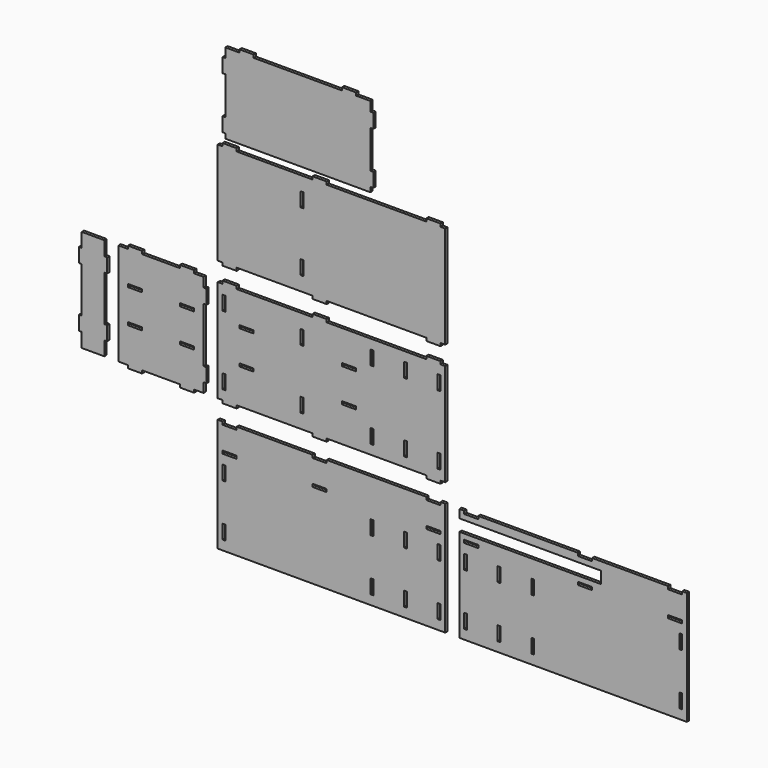
from build123d import *

# Parameters (mm, degrees)
F0_W     = 15.494
F0_H     = 76.2
F0_W_2   = 76.2
F0_H_2   = 15.494
F1_DEPTH = 15.494


# Not quite as in the source:
# - a feature names something its author has since deleted; it is built from what else it names


with BuildPart() as f1:
    # F0 (on Front) → F1 (new body)
    with BuildSketch(Plane.XZ):
        Polygon((1909.7625, -985.8375), (1909.7625, -376.2375), (1884.3625, -376.2375), (1884.3625, -391.7315), (1808.1625, -391.7315), (1808.1625, -376.2375), (1400.175, -376.2375), (1400.175, -391.7315), (1323.975, -391.7315), (1323.975, -376.2375), (788.9875, -376.2375), (788.9875, -391.7315), (712.7875, -391.7315), (712.7875, -376.2375), (687.3875, -376.2375), (687.3875, -420.6875), (1449.3875, -420.6875), (1449.3875, -484.1875), (687.3875, -484.1875), (687.3875, -985.8375), align=None)
        with Locations((720.5345, -896.9375)):
            Rectangle(F0_W, F0_H, mode=Mode.SUBTRACT)
        with Locations((901.1285, -896.9375)):
            Rectangle(F0_W, F0_H, mode=Mode.SUBTRACT)
        with Locations((1081.7225, -896.9375)):
            Rectangle(F0_W, F0_H, mode=Mode.SUBTRACT)
        with Locations((720.5345, -617.5375)):
            Rectangle(F0_W, F0_H, mode=Mode.SUBTRACT)
        with Locations((901.1285, -617.5375)):
            Rectangle(F0_W, F0_H, mode=Mode.SUBTRACT)
        with Locations((1081.7225, -617.5375)):
            Rectangle(F0_W, F0_H, mode=Mode.SUBTRACT)
        with Locations((750.8875, -520.8905)):
            Rectangle(F0_W_2, F0_H_2, mode=Mode.SUBTRACT)
        with Locations((1876.6155, -896.9375)):
            Rectangle(F0_W, F0_H, mode=Mode.SUBTRACT)
        with Locations((1362.075, -520.8905)):
            Rectangle(F0_W_2, F0_H_2, mode=Mode.SUBTRACT)
        with Locations((1876.6155, -617.5375)):
            Rectangle(F0_W, F0_H, mode=Mode.SUBTRACT)
        with Locations((1846.2625, -520.8905)):
            Rectangle(F0_W_2, F0_H_2, mode=Mode.SUBTRACT)
    extrude(amount=F1_DEPTH)


with BuildPart() as f1b:
    # F0 (on Front) → F1, piece 2 (new body)
    with BuildSketch(Plane.XZ):
        Polygon((-585.7875, -376.2375), (-611.1875, -376.2375), (-611.1875, -985.8375), (611.1875, -985.8375), (611.1875, -376.2375), (585.7875, -376.2375), (585.7875, -391.7315), (509.5875, -391.7315), (509.5875, -376.2375), (-25.4, -376.2375), (-25.4, -391.7315), (-101.6, -391.7315), (-101.6, -376.2375), (-509.5875, -376.2375), (-509.5875, -391.7315), (-585.7875, -391.7315), align=None)
        with Locations((-578.0405, -896.9375)):
            Rectangle(F0_W, F0_H, mode=Mode.SUBTRACT)
        with Locations((-578.0405, -617.5375)):
            Rectangle(F0_W, F0_H, mode=Mode.SUBTRACT)
        with Locations((-547.6875, -520.8905)):
            Rectangle(F0_W_2, F0_H_2, mode=Mode.SUBTRACT)
        with Locations((216.8525, -896.9375)):
            Rectangle(F0_W, F0_H, mode=Mode.SUBTRACT)
        with Locations((216.8525, -617.5375)):
            Rectangle(F0_W, F0_H, mode=Mode.SUBTRACT)
        with Locations((-63.5, -520.8905)):
            Rectangle(F0_W_2, F0_H_2, mode=Mode.SUBTRACT)
        with Locations((397.4465, -896.9375)):
            Rectangle(F0_W, F0_H, mode=Mode.SUBTRACT)
        with Locations((578.0405, -896.9375)):
            Rectangle(F0_W, F0_H, mode=Mode.SUBTRACT)
        with Locations((397.4465, -617.5375)):
            Rectangle(F0_W, F0_H, mode=Mode.SUBTRACT)
        with Locations((578.0405, -617.5375)):
            Rectangle(F0_W, F0_H, mode=Mode.SUBTRACT)
        with Locations((547.6875, -520.8905)):
            Rectangle(F0_W_2, F0_H_2, mode=Mode.SUBTRACT)
    extrude(amount=F1_DEPTH)


with BuildPart() as f1c:
    # F0 (on Front) → F1, piece 3 (new body)
    with BuildSketch(Plane.XZ):
        Polygon((585.7875, 376.2375), (611.1875, 376.2375), (611.1875, 925.5125), (585.7875, 925.5125), (509.5875, 925.5125), (-25.4, 925.5125), (-101.6, 925.5125), (-509.5875, 925.5125), (-585.7875, 925.5125), (-611.1875, 925.5125), (-611.1875, 376.2375), (-585.7875, 376.2375), (-509.5875, 376.2375), (-101.6, 376.2375), (-25.4, 376.2375), (509.5875, 376.2375), align=None)
        with Locations((-158.5595, 490.5375)):
            Rectangle(F0_W, F0_H, mode=Mode.SUBTRACT)
        with Locations((-158.5595, 811.2125)):
            Rectangle(F0_W, F0_H, mode=Mode.SUBTRACT)
        with Locations((-547.6875, 368.4905)):
            Rectangle(F0_W_2, F0_H_2)
        with Locations((-63.5, 368.4905)):
            Rectangle(F0_W_2, F0_H_2)
        with Locations((547.6875, 368.4905)):
            Rectangle(F0_W_2, F0_H_2)
        with Locations((547.6875, 933.2595)):
            Rectangle(F0_W_2, F0_H_2)
        with Locations((-63.5, 933.2595)):
            Rectangle(F0_W_2, F0_H_2)
        with Locations((-547.6875, 933.2595)):
            Rectangle(F0_W_2, F0_H_2)
    extrude(amount=F1_DEPTH)


with BuildPart() as f1d:
    # F0 (on Front) → F1, piece 4 (new body)
    with BuildSketch(Plane.XZ):
        Polygon((611.1875, -274.6375), (611.1875, 274.6375), (585.7875, 274.6375), (509.5875, 274.6375), (-25.4, 274.6375), (-101.6, 274.6375), (-509.5875, 274.6375), (-585.7875, 274.6375), (-611.1875, 274.6375), (-611.1875, -274.6375), (-585.7875, -274.6375), (-509.5875, -274.6375), (-101.6, -274.6375), (-25.4, -274.6375), (509.5875, -274.6375), (585.7875, -274.6375), align=None)
        with Locations((-578.0405, -185.7375)):
            Rectangle(F0_W, F0_H, mode=Mode.SUBTRACT)
        with Locations((-578.0405, 185.7375)):
            Rectangle(F0_W, F0_H, mode=Mode.SUBTRACT)
        with Locations((-158.5595, -160.3375)):
            Rectangle(F0_W, F0_H, mode=Mode.SUBTRACT)
        with Locations((216.8525, -185.7375)):
            Rectangle(F0_W, F0_H, mode=Mode.SUBTRACT)
        with Locations((-455.9935, -78.8035)):
            Rectangle(F0_W_2, F0_H_2, mode=Mode.SUBTRACT)
        with Locations((-455.9935, 101.7905)):
            Rectangle(F0_W_2, F0_H_2, mode=Mode.SUBTRACT)
        with Locations((-158.5595, 160.3375)):
            Rectangle(F0_W, F0_H, mode=Mode.SUBTRACT)
        with Locations((94.8055, -78.8035)):
            Rectangle(F0_W_2, F0_H_2, mode=Mode.SUBTRACT)
        with Locations((94.8055, 101.7905)):
            Rectangle(F0_W_2, F0_H_2, mode=Mode.SUBTRACT)
        with Locations((216.8525, 185.7375)):
            Rectangle(F0_W, F0_H, mode=Mode.SUBTRACT)
        with Locations((397.4465, -185.7375)):
            Rectangle(F0_W, F0_H, mode=Mode.SUBTRACT)
        with Locations((578.0405, -185.7375)):
            Rectangle(F0_W, F0_H, mode=Mode.SUBTRACT)
        with Locations((397.4465, 185.7375)):
            Rectangle(F0_W, F0_H, mode=Mode.SUBTRACT)
        with Locations((578.0405, 185.7375)):
            Rectangle(F0_W, F0_H, mode=Mode.SUBTRACT)
        with Locations((-547.6875, -282.3845)):
            Rectangle(F0_W_2, F0_H_2)
        with Locations((-63.5, -282.3845)):
            Rectangle(F0_W_2, F0_H_2)
        with Locations((-547.6875, 282.3845)):
            Rectangle(F0_W_2, F0_H_2)
        with Locations((-63.5, 282.3845)):
            Rectangle(F0_W_2, F0_H_2)
        with Locations((547.6875, 282.3845)):
            Rectangle(F0_W_2, F0_H_2)
        with Locations((547.6875, -282.3845)):
            Rectangle(F0_W_2, F0_H_2)
    extrude(amount=F1_DEPTH)


with BuildPart() as f1e:
    # F0 (on Front) → F1, piece 5 (new body)
    with BuildSketch(Plane.XZ):
        Polygon((-687.3875, 223.8375), (-687.3875, 274.6375), (-738.1875, 274.6375), (-814.3875, 274.6375), (-1017.5875, 274.6375), (-1093.7875, 274.6375), (-1144.5875, 274.6375), (-1144.5875, -274.6375), (-1093.7875, -274.6375), (-1017.5875, -274.6375), (-814.3875, -274.6375), (-738.1875, -274.6375), (-687.3875, -274.6375), (-687.3875, -223.8375), (-687.3875, -147.6375), (-687.3875, 147.6375), align=None)
        with Locations((-1055.6875, -78.8035)):
            Rectangle(F0_W_2, F0_H_2, mode=Mode.SUBTRACT)
        with Locations((-1055.6875, 101.7905)):
            Rectangle(F0_W_2, F0_H_2, mode=Mode.SUBTRACT)
        with Locations((-776.2875, -78.8035)):
            Rectangle(F0_W_2, F0_H_2, mode=Mode.SUBTRACT)
        with Locations((-776.2875, 101.7905)):
            Rectangle(F0_W_2, F0_H_2, mode=Mode.SUBTRACT)
        with Locations((-679.6405, -185.7375)):
            Rectangle(F0_W, F0_H)
        with Locations((-776.2875, -282.3845)):
            Rectangle(F0_W_2, F0_H_2)
        with Locations((-1055.6875, -282.3845)):
            Rectangle(F0_W_2, F0_H_2)
        with Locations((-1055.6875, 282.3845)):
            Rectangle(F0_W_2, F0_H_2)
        with Locations((-776.2875, 282.3845)):
            Rectangle(F0_W_2, F0_H_2)
        with Locations((-679.6405, 185.7375)):
            Rectangle(F0_W, F0_H)
    extrude(amount=F1_DEPTH)


with BuildPart() as f1f:
    # F0 (on Front) → F1, piece 6 (new body)
    with BuildSketch(Plane.XZ):
        Polygon((-1342.1995, -274.6375), (-1220.7875, -274.6375), (-1220.7875, -198.4375), (-1220.7875, -122.2375), (-1220.7875, 122.2375), (-1220.7875, 198.4375), (-1220.7875, 274.6375), (-1342.1995, 274.6375), (-1342.1995, 198.4375), (-1342.1995, 122.2375), (-1342.1995, -122.2375), (-1342.1995, -198.4375), align=None)
        with Locations((-1349.9465, 160.3375)):
            Rectangle(F0_W, F0_H)
        with Locations((-1213.0405, 160.3375)):
            Rectangle(F0_W, F0_H)
        with Locations((-1213.0405, -160.3375)):
            Rectangle(F0_W, F0_H)
        with Locations((-1349.9465, -160.3375)):
            Rectangle(F0_W, F0_H)
    extrude(amount=F1_DEPTH)


with BuildPart() as f1g:
    # F0 (on Front) → F1, piece 7 (new body)
    with BuildSketch(Plane.XZ):
        Polygon((-570.2935, 991.8065), (-570.2935, 966.4065), (209.1055, 966.4065), (209.1055, 991.8065), (209.1055, 1068.0065), (209.1055, 1271.2065), (209.1055, 1347.4065), (209.1055, 1398.2065), (132.9055, 1398.2065), (56.7055, 1398.2065), (-417.8935, 1398.2065), (-494.0935, 1398.2065), (-570.2935, 1398.2065), (-570.2935, 1347.4065), (-570.2935, 1271.2065), (-570.2935, 1068.0065), align=None)
        with Locations((-455.9935, 1405.9535)):
            Rectangle(F0_W_2, F0_H_2)
        with Locations((-578.0405, 1309.3065)):
            Rectangle(F0_W, F0_H)
        with Locations((-578.0405, 1029.9065)):
            Rectangle(F0_W, F0_H)
        with Locations((94.8055, 1405.9535)):
            Rectangle(F0_W_2, F0_H_2)
        with Locations((216.8525, 1309.3065)):
            Rectangle(F0_W, F0_H)
        with Locations((216.8525, 1029.9065)):
            Rectangle(F0_W, F0_H)
    extrude(amount=F1_DEPTH)


solid = Compound([f1.part, f1b.part, f1c.part, f1d.part, f1e.part, f1f.part, f1g.part])
